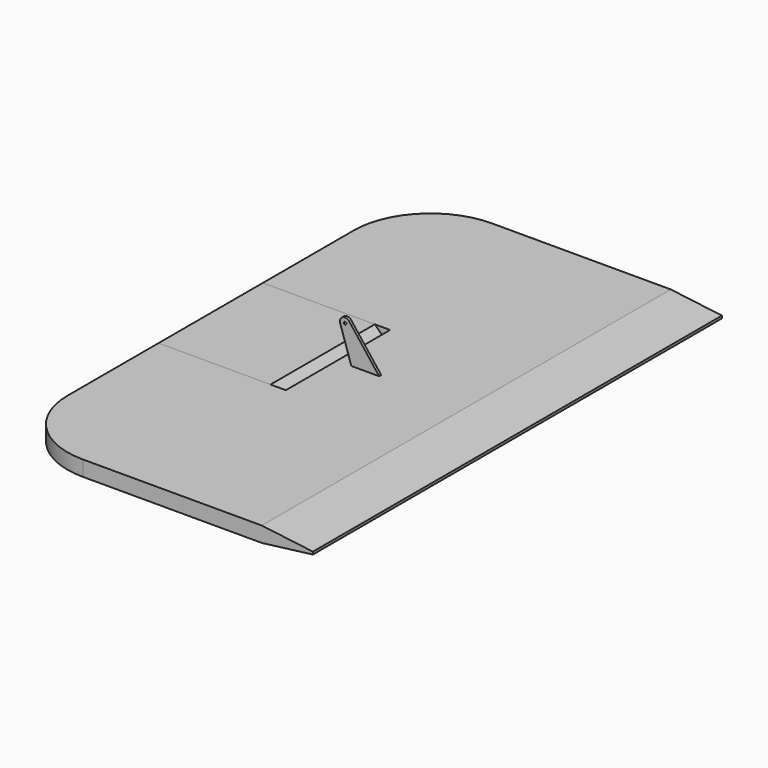
from build123d import *

# Parameters (mm, degrees)
F1_DEPTH = 6
F2_SIZE2 = 20
F2_SIZE  = 2.5
F3_DEPTH = 6
F4_SIZE2 = 3
F4_SIZE  = 3
F5_SIZE2 = 3
F5_SIZE  = 3
F6_SIZE2 = 2.99999
F6_SIZE  = 2.99999
F7_R     = 0.5
F8_DEPTH = 0.5


# Not quite as in the source:
# - a fillet or chamfer is up to 0.001 mm smaller than in the source, because OpenCascade refuses the exact size


with BuildPart() as f1:
    # F0 (on Top) → F1 (new body)
    with BuildSketch(Plane.XY):
        with BuildLine():
            Line((61.5713464236, -100), (61.5713464236, 100))
            Line((61.5713464236, 100), (-28.4286535764, 100))
            ThreePointArc((-28.4286535764, 100), (-49.641857012, 91.2132034356), (-58.4286535764, 70))
            Line((-58.4286535764, 70), (-58.4286535764, 25.5028065294))
            Line((-58.4286535764, 25.5028065294), (-11.6032855585, 25.5028065294))
            Line((-11.6032855585, 25.5028065294), (-11.6032855585, 0))
            Line((-11.6032855585, 0), (-11.6032855585, -25.5028065294))
            Line((-11.6032855585, -25.5028065294), (-58.4286535764, -25.5028065294))
            Line((-58.4286535764, -25.5028065294), (-58.4286535764, -70))
            ThreePointArc((-58.4286535764, -70), (-49.641857012, -91.2132034356), (-28.4286535764, -100))
            Line((-28.4286535764, -100), (61.5713464236, -100))
        make_face()
    extrude(amount=F1_DEPTH)

    # F2
    f2_edges = [f1.edges().sort_by_distance(p)[0] for p in [
        (61.571346, 0, 6),
        (61.571346, 0, 0),
    ]]
    f2_side = f1.faces().sort_by_distance((61.571346, 0, 3))[0]
    chamfer(f2_edges, length=F2_SIZE, length2=F2_SIZE2, reference=f2_side)

    # F4
    f4_edges = [f1.edges().sort_by_distance(p)[0] for p in [
        (-11.603286, 0, 6),
    ]]
    chamfer(f4_edges, length=F4_SIZE, length2=F4_SIZE2)

    # F6 (size 3 and 3 in the source; OpenCascade refuses exactly that, so slightly less here)
    f6_edges = [f1.edges().sort_by_distance(p)[0] for p in [
        (-11.603286, 0, 0),
    ]]
    chamfer(f6_edges, length=F6_SIZE, length2=F6_SIZE2)

    # F7 (on Front) → F8 (join, symmetric)
    with BuildSketch(Plane.XZ):
        with BuildLine():
            Line((-7.3477944259, 19.2926249586), (-2.9993071221, 6))
            Line((-2.9993071221, 6), (7.8871631995, 6))
            Line((7.8871631995, 6), (-3.8671067929, 21.1409176701))
            ThreePointArc((-3.8671067929, 21.1409176701), (-3.5548827609, 20.5626830442), (-3.4469229787, 19.9144671741))
            ThreePointArc((-3.4469229787, 19.9144671741), (-5.1320761068, 17.9394047834), (-7.3477944259, 19.2926249586))
        make_face()
        with BuildLine():
            ThreePointArc((-3.8671067929, 21.1409176701), (-6.3849078437, 21.6808715426), (-7.3477944259, 19.2926249586))
            ThreePointArc((-7.3477944259, 19.2926249586), (-5.1320761068, 17.9394047834), (-3.4469229787, 19.9144671741))
            ThreePointArc((-3.4469229787, 19.9144671741), (-3.5548827609, 20.5626830442), (-3.8671067929, 21.1409176701))
        make_face()
        with Locations((-5.4469229787, 19.9144671741)):
            Circle(F7_R, mode=Mode.SUBTRACT)
    extrude(amount=F8_DEPTH, both=True)


with BuildPart() as f3:
    # F0 (on Top) → F3 (new body)
    with BuildSketch(Plane.XY):
        Polygon((-11.6032855585, 25.5028065294), (-58.4286535764, 25.5028065294), (-58.4286535764, 0), (-58.4286535764, -25.5028065294), (-11.6032855585, -25.5028065294), (-11.6032855585, 0), align=None)
    extrude(amount=F3_DEPTH)

    # F5
    f5_edges = [f3.edges().sort_by_distance(p)[0] for p in [
        (-11.603286, 0, 6),
    ]]
    chamfer(f5_edges, length=F5_SIZE, length2=F5_SIZE2)


solid = Compound([f1.part, f3.part])
